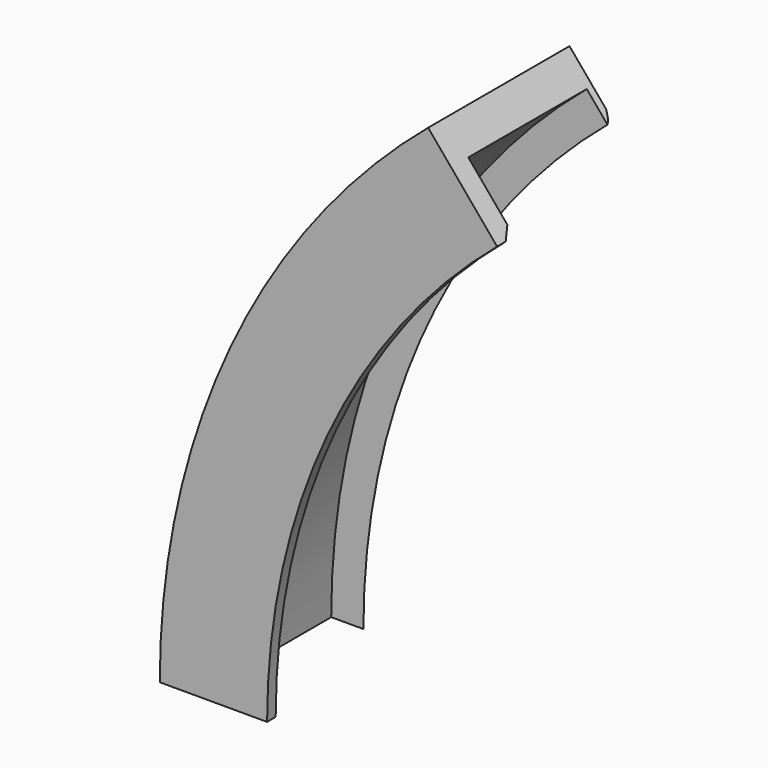
from build123d import *

# Parameters (mm, degrees)
F1_ANGLE    = 50
F2_SIZE     = 1.5
F3_T2_ANGLE = 53.1281028161


# Not quite as in the source:
# - a fillet or chamfer that OpenCascade refuses, or shapes differently, is made with other operations: its cross-section is extruded or revolved along the edge and cut away or added


with BuildPart() as f1:
    # F0 (on Top) → F1 (revolve)
    with BuildSketch(Plane.XY):
        Polygon((-90, -10), (-100, -10), (-100, 10.7), (-95, 10.7), (-97, 11.7), (-105, 11.7), (-105, -13), (-90, -13), align=None)
    revolve(axis=Axis((0, 3.89609579, 0), (0, 1, 0)), revolution_arc=F1_ANGLE)

    # F2
    f2_edges = [f1.edges().sort_by_distance(p)[0] for p in [
        (-81.567701, -10, 38.035644),
    ]]
    chamfer(f2_edges, length=F2_SIZE)

    # F3: chamfer of 1 x 0.5 on 1 edges, made by hand

    # F3_s1 → F3_t2 (revolve, cut)
    with BuildSketch(Plane(origin=(0, 0, 0), x_dir=(0, 1, 0), z_dir=(0.0272944566, 0, -0.9996274369))):
        Polygon((10.7, -95.5), (11.1472135955, -95.894427191), (10.7, -95), align=None)
    revolve(axis=Axis((0, 10.7, 0), (0, 1, 0)), revolution_arc=F3_T2_ANGLE, mode=Mode.SUBTRACT)


solid = f1.part
